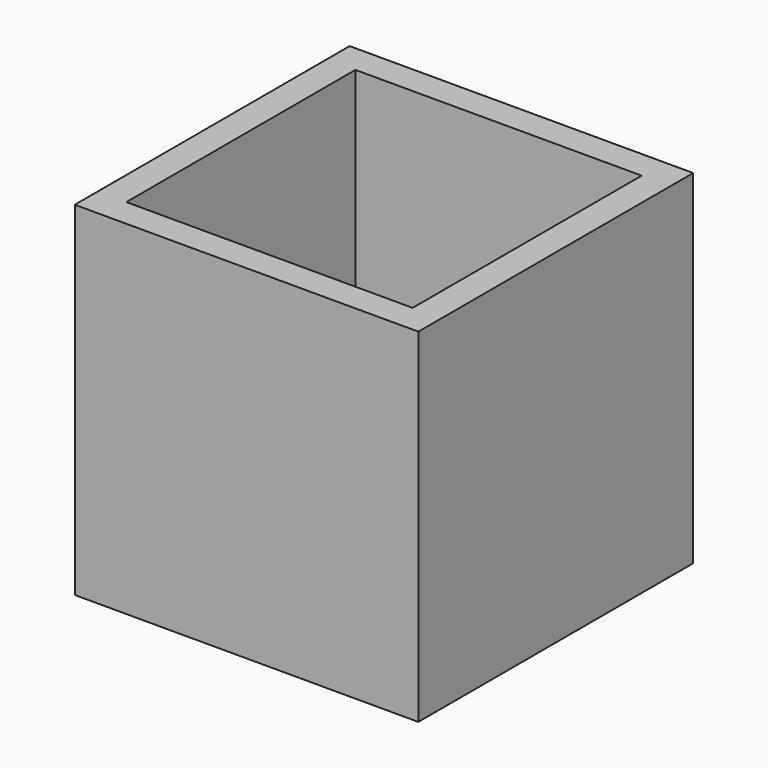
from build123d import *

# Parameters (mm, degrees)
F1_W     = 152.4
F1_H     = 152.4
F1_W_2   = 127
F1_H_2   = 127
F2_DEPTH = 152.4


# Not quite as in the source:
# - a variable given as a bare number and used for a length is read in inches; the dataset says mm whatever the document's units were


with BuildPart() as f2:
    # F1 (on Top) → F2 (new body)
    with BuildSketch(Plane.XY):
        with Locations((0.3060060553, 7.9399240886)):
            Rectangle(F1_W, F1_H)
        with Locations((0.3060060553, 7.9399240886)):
            Rectangle(F1_W_2, F1_H_2, mode=Mode.SUBTRACT)
    extrude(amount=F2_DEPTH)


solid = f2.part
